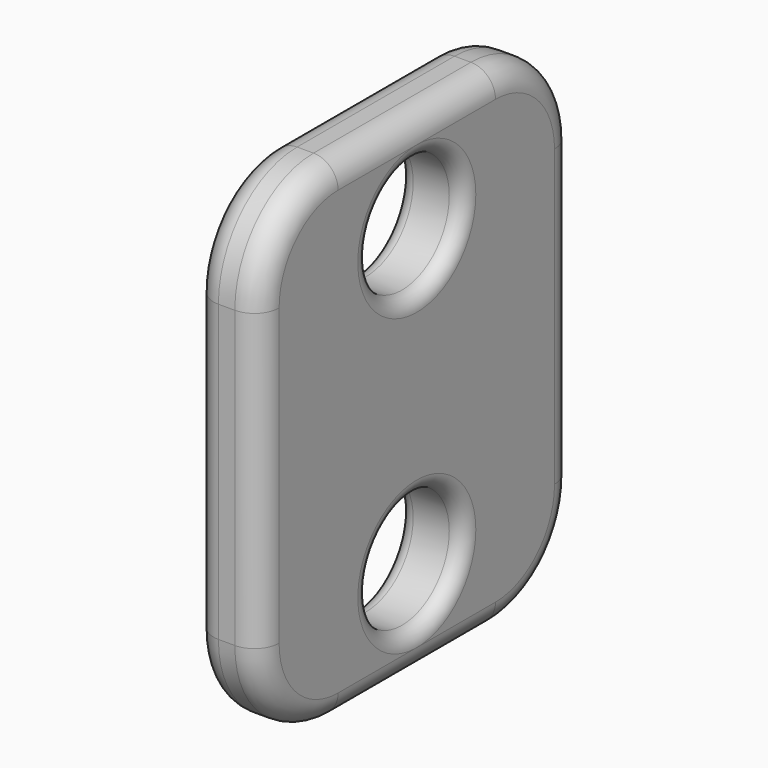
from build123d import *

# Parameters (mm, degrees)
F1_DEPTH = 40
F2_R     = 6
F3_DEPTH = 25
F4_R     = 10
F5_R     = 2.5
F6_R     = 1.49999


# Not quite as in the source:
# - a fillet or chamfer is up to 0.001 mm smaller than in the source, because OpenCascade refuses the exact size
# - a feature names something its author has since deleted; it is built from what else it names


with BuildPart() as f1:
    # F0 (on Front) → F1 (new body)
    with BuildSketch(Plane.XZ):
        Polygon((-3.34, 19.1122043878), (-3.34, -0.8877956122), (-3.34, -30.8877956122), (3.33, -30.8877956122), (3.33, -0.8877956122), (3.33, 13.6661529541), (3.33, 19.1122043878), align=None)
    extrude(amount=F1_DEPTH)

    # F2 (on face) → F3 (cut)
    with BuildSketch(Plane.YZ.offset(3.33)):
        with Locations((-20, 9.1122043878)):
            Circle(F2_R)
        with Locations((-20, -20.8877956122)):
            Circle(F2_R)
    extrude(amount=-F3_DEPTH, mode=Mode.SUBTRACT)

    # F4
    f4_edges = [f1.edges().sort_by_distance(p)[0] for p in [
        (-0.005, -40, 19.112204),
        (-0.005, 0, 19.112204),
        (-0.005, 0, -30.887796),
        (-0.005, -40, -30.887796),
    ]]
    fillet(f4_edges, radius=F4_R)

    # F5
    f5_edges = [f1.edges().sort_by_distance(p)[0] for p in [
        (3.33, -20, 19.112204),
        (-3.34, -20, -30.887796),
        (-3.34, -20, 19.112204),
        (-3.34, -37.071068, 16.183272),
        (-3.34, -40, -5.887796),
        (-3.34, -37.071068, -27.958863),
        (-3.34, -2.928932, -27.958863),
        (-3.34, -2.928932, 16.183272),
        (-3.34, 0, -5.887796),
    ]]
    fillet(f5_edges, radius=F5_R)

    # F6 (radius 1.5 in the source; OpenCascade refuses exactly that, so slightly less here)
    f6_edges = [f1.edges().sort_by_distance(p)[0] for p in [
        (3.33, -26, 9.112204),
        (-0.005, -14, 9.112204),
        (-3.34, -26, 9.112204),
        (3.33, -26, -20.887796),
        (-3.34, -26, -20.887796),
    ]]
    fillet(f6_edges, radius=F6_R)


solid = f1.part
